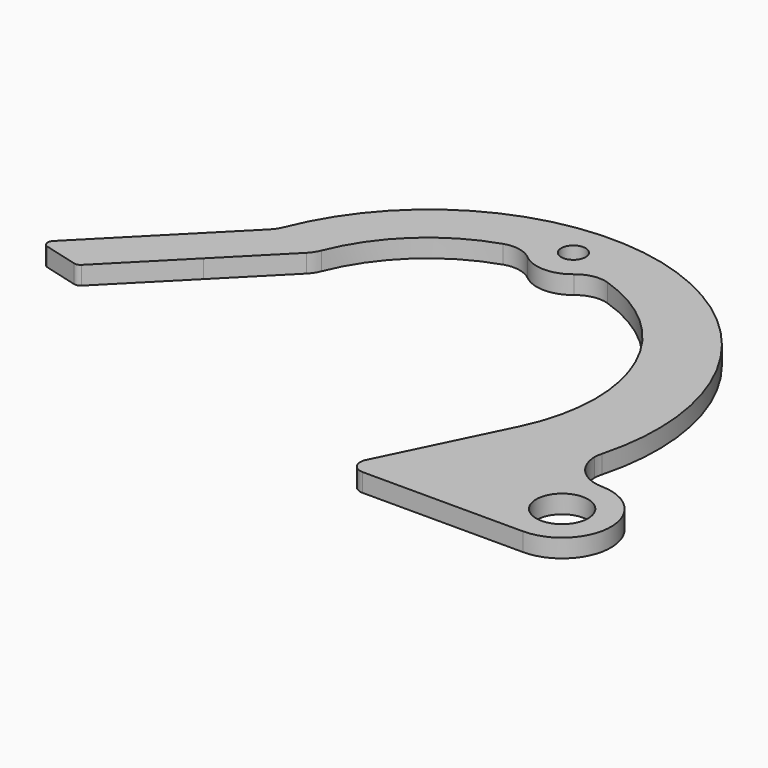
from build123d import *

# Parameters (mm, degrees)
F0_R        = 2
F0_R_2      = 4.25
F1_DEPTH    = 3
F2_R        = 5
F3_T1_DEPTH = 3
F4_R        = 1


# Not quite as in the source:
# - a fillet or chamfer that OpenCascade refuses, or shapes differently, is made with other operations: its cross-section is extruded or revolved along the edge and cut away or added


with BuildPart() as f1:
    # F0 (on Top) → F1 (new body)
    with BuildSketch(Plane.XY):
        with BuildLine():
            Line((-61.2338289806, 21.9643939736), (-49.74418384, 33.565422262))
            ThreePointArc((-49.74418384, 33.565422262), (-49.1122742467, 39.7914012722), (-47.4538011201, 45.8256030636))
            Line((-47.4538011201, 45.8256030636), (-69.0197217506, 24.0506176536))
            Line((-69.0197217506, 24.0506176536), (-61.2338289806, 21.9643939736))
        make_face()
        with BuildLine():
            ThreePointArc((-47.4538011201, 45.8256030636), (-49.1122742467, 39.7914012722), (-49.74418384, 33.565422262))
            Line((-49.74418384, 33.565422262), (-39.66790835, 43.7393793835))
            ThreePointArc((-39.66790835, 43.7393793835), (-31.7050161187, 55.3610537789), (-19.0319758246, 61.5145095676))
            ThreePointArc((-19.0319758246, 61.5145095676), (-19.0541360585, 67.1935796255), (-14.3311022775, 70.3471933782))
            ThreePointArc((-14.3311022775, 70.3471933782), (-34.5629581909, 63.0443589232), (-47.4538011201, 45.8256030636))
        make_face()
        with BuildLine():
            ThreePointArc((-13.7575576035, 70.3746690788), (-14.04438253, 70.3620290137), (-14.3311022775, 70.3471933782))
            ThreePointArc((-14.3311022775, 70.3471933782), (-19.0541360585, 67.1935796255), (-19.0319758246, 61.5145095676))
            ThreePointArc((-19.0319758246, 61.5145095676), (-13.7575576035, 62.0250576942), (-8.4831393824, 61.5145095676))
            ThreePointArc((-8.4831393824, 61.5145095676), (-7.941781244, 62.8992893525), (-7.7575576035, 64.3746690788))
            ThreePointArc((-7.7575576035, 64.3746690788), (-9.5149169164, 68.6173097659), (-13.7575576035, 70.3746690788))
        make_face()
        with Locations((-13.7575576035, 64.3746690788)):
            Circle(F0_R, mode=Mode.SUBTRACT)
        with BuildLine():
            ThreePointArc((-8.4831393824, 61.5145095676), (-13.7575576035, 62.0250576942), (-19.0319758246, 61.5145095676))
            ThreePointArc((-19.0319758246, 61.5145095676), (-13.7575576035, 58.3746690788), (-8.4831393824, 61.5145095676))
        make_face()
        with BuildLine():
            ThreePointArc((1.4030809655, 2.8767422936), (1.5045728658, 0.9401614715), (3.2006690581, 0))
            Line((3.2006690581, 0), (5.7364393854, 0))
            ThreePointArc((5.7364393854, 0), (16.9754981283, 9.4077450038), (23.75, 22.4049843981))
            ThreePointArc((23.75, 22.4049843981), (24.8731060123, 27.6016835392), (25.25, 32.9049843981))
            ThreePointArc((25.25, 32.9049843981), (13.7280348551, 59.9492389647), (-13.7575576035, 70.3746690788))
            ThreePointArc((-13.7575576035, 70.3746690788), (-9.5149169164, 68.6173097659), (-7.7575576035, 64.3746690788))
            ThreePointArc((-7.7575576035, 64.3746690788), (-7.941781244, 62.8992893525), (-8.4831393824, 61.5145095676))
            ThreePointArc((-8.4831393824, 61.5145095676), (7.4709197451, 52.0065264385), (13.7424423965, 34.5250576942))
            ThreePointArc((13.7424423965, 34.5250576942), (13.0376191781, 28.3389036997), (10.9592786697, 22.4698511575))
            Line((10.9592786697, 22.4698511575), (1.4030809655, 2.8767422936))
        make_face()
        with BuildLine():
            ThreePointArc((23.75, 22.4049843981), (16.9754981283, 9.4077450038), (5.7364393854, 0))
            Line((5.7364393854, 0), (29.5, 0))
            ThreePointArc((29.5, 0), (37.5, 8), (29.5, 16))
            Line((29.5, 16), (23.75, 16))
            Line((23.75, 16), (23.75, 22.4049843981))
        make_face()
        with Locations((29.5, 8)):
            Circle(F0_R_2, mode=Mode.SUBTRACT)
    extrude(amount=F1_DEPTH)

    # F2
    f2_edges = [f1.edges().sort_by_distance(p)[0] for p in [
        (-19.031976, 61.51451, 1.5),
        (-8.483139, 61.51451, 1.5),
        (-39.667908, 43.739379, 1.5),
        (-47.453801, 45.825603, 1.5),
    ]]
    fillet(f2_edges, radius=F2_R)

    # F3: fillet of radius 6 on 2 edges, made by hand

    # F3_s2 → F3_t1 (join)
    with BuildSketch(Plane.XY):
        with BuildLine():
            ThreePointArc((23.9568965517, 23.1422674559), (23.8019490297, 22.3680713423), (23.75, 21.5802327452))
            Line((23.75, 21.5802327452), (23.75, 22.4049843981))
            ThreePointArc((23.75, 22.4049843981), (23.8553302711, 22.773097801), (23.9568965517, 23.1422674559))
        make_face()
        with BuildLine():
            ThreePointArc((23.75, 21.9977676792), (25.4696462095, 17.7931783498), (29.6428571429, 15.9987243881))
            Line((29.6428571429, 15.9987243881), (29.6321428571, 15.398820059))
            ThreePointArc((29.6321428571, 15.398820059), (29.5, 15.4), (23.75, 15.4))
            Line((23.75, 15.4), (23.15, 16))
            Line((23.15, 16), (23.15, 21.9977676792))
            Line((23.15, 21.9977676792), (23.75, 21.9977676792))
        make_face()
    extrude(amount=F3_T1_DEPTH)

    # F4
    f4_edges = [f1.edges().sort_by_distance(p)[0] for p in [
        (-69.019722, 24.050618, 1.5),
        (-61.233829, 21.964394, 1.5),
    ]]
    fillet(f4_edges, radius=F4_R)


solid = f1.part
